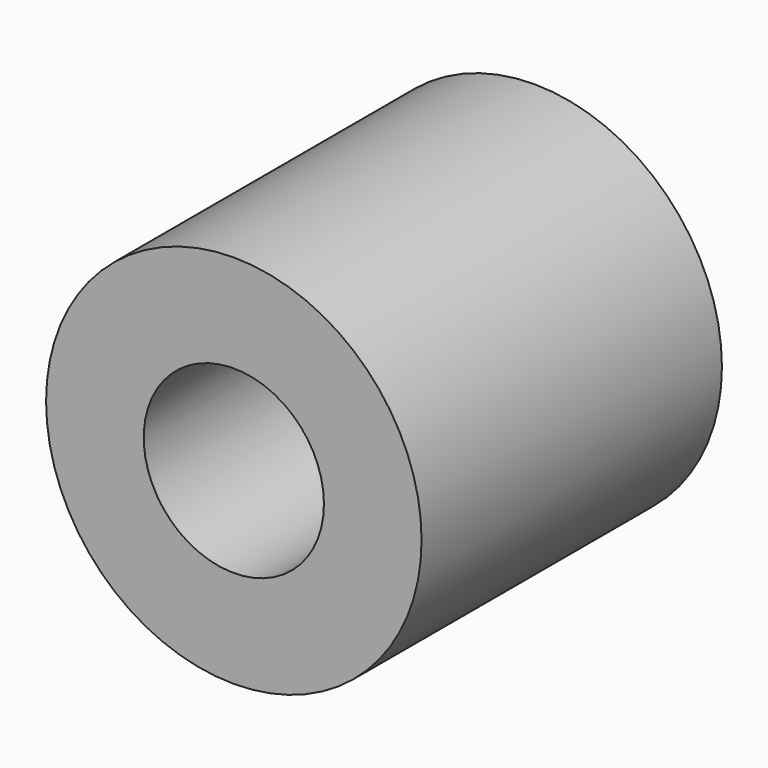
from build123d import *

# Parameters (mm, degrees)
F1_R     = 12.5
F1_R_2   = 6
F2_DEPTH = 25


# Not quite as in the source:
# - a feature names something its author has since deleted; it is built from what else it names


with BuildPart() as f2:
    # F1 (on Front) → F2 (new body)
    with BuildSketch(Plane.XZ):
        Circle(F1_R)
        Circle(F1_R_2, mode=Mode.SUBTRACT)
    extrude(amount=-F2_DEPTH)


solid = f2.part
